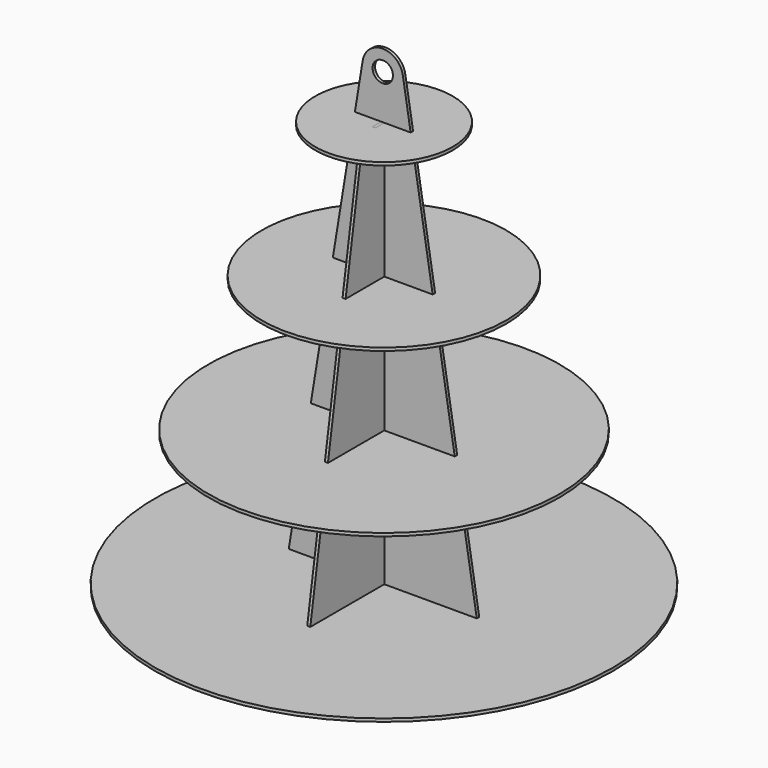
from build123d import *

# Parameters (mm, degrees)
F0_R      = 10
F1_DEPTH  = 1.5
F2_W      = 3
F2_H      = 220
F3_DEPTH  = 25
F5_DEPTH  = 1.5
F6_W      = 3
F6_H      = 212
F7_DEPTH  = 12.5
F9_R      = 225
F10_DEPTH = 3
F12_R     = 172.5
F13_DEPTH = 3
F15_R     = 120
F16_DEPTH = 3
F18_R     = 67.5
F19_DEPTH = 3


with BuildPart() as f1:
    # F0 (on Front) → F1 (new body, symmetric)
    with BuildSketch(Plane.XZ):
        with BuildLine():
            Line((-92.3427922293, 30), (-195, 30))
            add(Edge.make_bspline(
                [(-195, 30), (-195, 16.186110581), (-168.2676257137, 15.093790554), (-141.795995516, 15.0074163979)],
                knots=[0, 0, 0, 0, 56.9561251752, 56.9561251752, 56.9561251752, 56.9561251752], degree=3))
            ThreePointArc((-141.795995516, 15.0074163979), (-137.776195244, 12.9586763901), (-137.0427819368, 8.5069087898))
            Line((-137.0427819368, 8.5069087898), (-139.3101033649, 1.3001068448))
            ThreePointArc((-139.3101033649, 1.3001068448), (-139.1624566765, 0.4084371736), (-138.3561977712, 0))
            Line((-138.3561977712, 0), (0, 0))
            Line((0, 0), (138.3561977712, 0))
            ThreePointArc((138.3561977712, 0), (139.1624566765, 0.4084371736), (139.3101033649, 1.3001068448))
            Line((139.3101033649, 1.3001068448), (137.0427819368, 8.5069087898))
            ThreePointArc((137.0427819368, 8.5069087898), (137.776195244, 12.9586763901), (141.795995516, 15.0074163979))
            add(Edge.make_bspline(
                [(195, 30), (195, 16.186110581), (168.2676257137, 15.093790554), (141.795995516, 15.0074163979)],
                knots=[0, 0, 0, 0, 56.9561251752, 56.9561251752, 56.9561251752, 56.9561251752], degree=3))
            Line((195, 30), (92.3427922293, 30))
            Line((92.3427922293, 30), (92.3427922293, 33))
            Line((92.3427922293, 33), (74.5588604965, 142.1962788761))
            ThreePointArc((74.5588604965, 142.1962788761), (75.6847331024, 146.2389345764), (79.4938409783, 148))
            Line((79.4938409783, 148), (82.5, 148))
            add(Edge.make_bspline(
                [(142.5, 163), (142.5, 151.0542502936), (110.9798626697, 148), (82.5, 148)],
                knots=[0, 0, 0, 0, 61.8465843843, 61.8465843843, 61.8465843843, 61.8465843843], degree=3))
            Line((142.5, 163), (70.6821372619, 163))
            Line((70.6821372619, 163), (70.6821372619, 166))
            Line((70.6821372619, 166), (52.7101309279, 276.3510879995))
            ThreePointArc((52.7101309279, 276.3510879995), (53.6868072822, 280.2096132801), (57.1717998525, 282.1323563276))
            add(Edge.make_bspline(
                [(90, 296), (90, 287.8812796125), (75.4408356741, 283.8695464407), (57.1717998525, 282.1323563276)],
                knots=[0, 0, 0, 0, 42.0329521278, 42.0329521278, 42.0329521278, 42.0329521278], degree=3))
            Line((90, 296), (49.0214822946, 296))
            Line((49.0214822946, 296), (49.0214822946, 299))
            Line((49.0214822946, 299), (29.5550758212, 418.5269517407))
            ThreePointArc((29.5550758212, 418.5269517407), (30.0968650968, 421.7181131313), (32.479761139, 423.9087416009))
            add(Edge.make_bspline(
                [(32.479761139, 423.9087416009), (25.3871356607, 420.7942687696), (11.9619410008, 419.2400986089), (0, 418.4677997632)],
                knots=[10.6465175628, 10.6465175628, 10.6465175628, 10.6465175628, 34.8130753377, 34.8130753377, 34.8130753377, 34.8130753377], degree=3))
            add(Edge.make_bspline(
                [(-32.479761139, 423.9087416009), (-25.3871356607, 420.7942687696), (-11.9619410008, 419.2400986089), (0, 418.4677997632)],
                knots=[10.6465175628, 10.6465175628, 10.6465175628, 10.6465175628, 34.8130753377, 34.8130753377, 34.8130753377, 34.8130753377], degree=3))
            ThreePointArc((-32.479761139, 423.9087416009), (-30.0968650968, 421.7181131313), (-29.5550758212, 418.5269517407))
            Line((-29.5550758212, 418.5269517407), (-49.0214822946, 299))
            Line((-49.0214822946, 299), (-49.0214822946, 296))
            Line((-49.0214822946, 296), (-90, 296))
            add(Edge.make_bspline(
                [(-90, 296), (-90, 287.8812796125), (-75.4408356741, 283.8695464407), (-57.1717998525, 282.1323563276)],
                knots=[0, 0, 0, 0, 42.0329521278, 42.0329521278, 42.0329521278, 42.0329521278], degree=3))
            ThreePointArc((-57.1717998525, 282.1323563276), (-53.6868072822, 280.2096132801), (-52.7101309279, 276.3510879995))
            Line((-52.7101309279, 276.3510879995), (-70.6821372619, 166))
            Line((-70.6821372619, 166), (-70.6821372619, 163))
            Line((-70.6821372619, 163), (-142.5, 163))
            add(Edge.make_bspline(
                [(-142.5, 163), (-142.5, 151.0542502936), (-110.9798626697, 148), (-82.5, 148)],
                knots=[0, 0, 0, 0, 61.8465843843, 61.8465843843, 61.8465843843, 61.8465843843], degree=3))
            Line((-82.5, 148), (-79.4938409783, 148))
            ThreePointArc((-79.4938409783, 148), (-75.6847331024, 146.2389345764), (-74.5588604965, 142.1962788761))
            Line((-74.5588604965, 142.1962788761), (-92.3427922293, 33))
            Line((-92.3427922293, 33), (-92.3427922293, 30))
        make_face()
        with BuildLine():
            add(Edge.make_bspline(
                [(-37.5, 429), (-37.5, 426.955715158), (-35.6043998411, 425.2808149431), (-32.479761139, 423.9087416009)],
                knots=[0, 0, 0, 0, 10.6465175628, 10.6465175628, 10.6465175628, 10.6465175628], degree=3))
            add(Edge.make_bspline(
                [(-32.479761139, 423.9087416009), (-25.3871356607, 420.7942687696), (-11.9619410008, 419.2400986089), (0, 418.4677997632)],
                knots=[10.6465175628, 10.6465175628, 10.6465175628, 10.6465175628, 34.8130753377, 34.8130753377, 34.8130753377, 34.8130753377], degree=3))
            add(Edge.make_bspline(
                [(32.479761139, 423.9087416009), (25.3871356607, 420.7942687696), (11.9619410008, 419.2400986089), (0, 418.4677997632)],
                knots=[10.6465175628, 10.6465175628, 10.6465175628, 10.6465175628, 34.8130753377, 34.8130753377, 34.8130753377, 34.8130753377], degree=3))
            add(Edge.make_bspline(
                [(37.5, 429), (37.5, 426.955715158), (35.6043998411, 425.2808149431), (32.479761139, 423.9087416009)],
                knots=[0, 0, 0, 0, 10.6465175628, 10.6465175628, 10.6465175628, 10.6465175628], degree=3))
            Line((37.5, 429), (27.3608273272, 429))
            Line((27.3608273272, 429), (27.3608273272, 432))
            Line((27.3608273272, 432), (19.7399219269, 478.793618188))
            ThreePointArc((19.7399219269, 478.793618188), (0, 495.5787336922), (-19.7399219269, 478.793618188))
            Line((-19.7399219269, 478.793618188), (-27.3608273272, 432))
            Line((-27.3608273272, 432), (-27.3608273272, 429))
            Line((-27.3608273272, 429), (-37.5, 429))
        make_face()
        with Locations((0, 475.5787336922)):
            Circle(F0_R, mode=Mode.SUBTRACT)
    extrude(amount=F1_DEPTH, both=True)

    # F2 (on face) → F3 (cut)
    with BuildSketch(Plane.XZ.offset(1.5)):
        with Locations((0, 110)):
            Rectangle(F2_W, F2_H)
    extrude(amount=-F3_DEPTH, mode=Mode.SUBTRACT)


with BuildPart() as f5:
    # F4 (on Right) → F5 (new body, symmetric)
    with BuildSketch(Plane.YZ):
        with BuildLine():
            Line((-92.3427922293, 30), (-195, 30))
            add(Edge.make_bspline(
                [(-195, 30), (-195, 16.335147151), (-168.5112592434, 15.1188411943), (-142.5647102575, 15.0105780321)],
                knots=[0, 0, 0, 0, 56.3416316551, 56.3416316551, 56.3416316551, 56.3416316551], degree=3))
            ThreePointArc((-142.5647102575, 15.0105780321), (-138.4043979513, 12.7524780168), (-137.991624861, 8.0368834052))
            Line((-137.991624861, 8.0368834052), (-140.631448797, 1.8925963671))
            ThreePointArc((-140.631448797, 1.8925963671), (-140.5487271046, 0.9492227505), (-139.7162225162, 0.4978550853))
            Line((-139.7162225162, 0.4978550853), (0, 0))
            Line((0, 0), (139.7162225162, 0.4978550853))
            ThreePointArc((139.7162225162, 0.4978550853), (140.5487271046, 0.9492227505), (140.631448797, 1.8925963671))
            Line((140.631448797, 1.8925963671), (137.991624861, 8.0368834052))
            ThreePointArc((137.991624861, 8.0368834052), (138.4043979513, 12.7524780168), (142.5647102575, 15.0105780321))
            add(Edge.make_bspline(
                [(195, 30), (195, 16.335147151), (168.5112592434, 15.1188411943), (142.5647102575, 15.0105780321)],
                knots=[0, 0, 0, 0, 56.3416316551, 56.3416316551, 56.3416316551, 56.3416316551], degree=3))
            Line((195, 30), (92.3427922293, 30))
            Line((92.3427922293, 30), (92.3427922293, 33))
            Line((92.3427922293, 33), (74.5588604965, 142.1962788761))
            ThreePointArc((74.5588604965, 142.1962788761), (75.6847331024, 146.2389345764), (79.4938409783, 148))
            Line((79.4938409783, 148), (82.5, 148))
            add(Edge.make_bspline(
                [(142.5, 163), (142.5, 151.0542502936), (110.9798626697, 148), (82.5, 148)],
                knots=[0, 0, 0, 0, 61.8465843843, 61.8465843843, 61.8465843843, 61.8465843843], degree=3))
            Line((142.5, 163), (70.6821372619, 163))
            Line((70.6821372619, 163), (70.6821372619, 166))
            Line((70.6821372619, 166), (52.7101309279, 276.3510879995))
            ThreePointArc((52.7101309279, 276.3510879995), (53.6868072822, 280.2096132801), (57.1717998525, 282.1323563276))
            add(Edge.make_bspline(
                [(90, 296), (90, 287.8812796125), (75.4408356741, 283.8695464407), (57.1717998525, 282.1323563276)],
                knots=[0, 0, 0, 0, 42.0329521278, 42.0329521278, 42.0329521278, 42.0329521278], degree=3))
            Line((90, 296), (49.0214822946, 296))
            Line((49.0214822946, 296), (49.0214822946, 299))
            Line((49.0214822946, 299), (29.5550758212, 418.5269517407))
            ThreePointArc((29.5550758212, 418.5269517407), (30.0968650968, 421.7181131313), (32.479761139, 423.9087416009))
            add(Edge.make_bspline(
                [(32.479761139, 423.9087416009), (25.3871356607, 420.7942687696), (11.9619410008, 419.2400986089), (0, 418.4677997632)],
                knots=[10.6465175628, 10.6465175628, 10.6465175628, 10.6465175628, 34.8130753377, 34.8130753377, 34.8130753377, 34.8130753377], degree=3))
            add(Edge.make_bspline(
                [(-32.479761139, 423.9087416009), (-25.3871356607, 420.7942687696), (-11.9619410008, 419.2400986089), (0, 418.4677997632)],
                knots=[10.6465175628, 10.6465175628, 10.6465175628, 10.6465175628, 34.8130753377, 34.8130753377, 34.8130753377, 34.8130753377], degree=3))
            ThreePointArc((-32.479761139, 423.9087416009), (-30.0968650968, 421.7181131313), (-29.5550758212, 418.5269517407))
            Line((-29.5550758212, 418.5269517407), (-49.0214822946, 299))
            Line((-49.0214822946, 299), (-49.0214822946, 296))
            Line((-49.0214822946, 296), (-90, 296))
            add(Edge.make_bspline(
                [(-90, 296), (-90, 287.8812796125), (-75.4408356741, 283.8695464407), (-57.1717998525, 282.1323563276)],
                knots=[0, 0, 0, 0, 42.0329521278, 42.0329521278, 42.0329521278, 42.0329521278], degree=3))
            ThreePointArc((-57.1717998525, 282.1323563276), (-53.6868072822, 280.2096132801), (-52.7101309279, 276.3510879995))
            Line((-52.7101309279, 276.3510879995), (-70.6821372619, 166))
            Line((-70.6821372619, 166), (-70.6821372619, 163))
            Line((-70.6821372619, 163), (-142.5, 163))
            add(Edge.make_bspline(
                [(-142.5, 163), (-142.5, 151.0542502936), (-110.9798626697, 148), (-82.5, 148)],
                knots=[0, 0, 0, 0, 61.8465843843, 61.8465843843, 61.8465843843, 61.8465843843], degree=3))
            Line((-82.5, 148), (-79.4938409783, 148))
            ThreePointArc((-79.4938409783, 148), (-75.6847331024, 146.2389345764), (-74.5588604965, 142.1962788761))
            Line((-74.5588604965, 142.1962788761), (-92.3427922293, 33))
            Line((-92.3427922293, 33), (-92.3427922293, 30))
        make_face()
        with BuildLine():
            add(Edge.make_bspline(
                [(-37.5, 429), (-37.5, 426.955715158), (-35.6043998411, 425.2808149431), (-32.479761139, 423.9087416009)],
                knots=[0, 0, 0, 0, 10.6465175628, 10.6465175628, 10.6465175628, 10.6465175628], degree=3))
            add(Edge.make_bspline(
                [(-32.479761139, 423.9087416009), (-25.3871356607, 420.7942687696), (-11.9619410008, 419.2400986089), (0, 418.4677997632)],
                knots=[10.6465175628, 10.6465175628, 10.6465175628, 10.6465175628, 34.8130753377, 34.8130753377, 34.8130753377, 34.8130753377], degree=3))
            add(Edge.make_bspline(
                [(32.479761139, 423.9087416009), (25.3871356607, 420.7942687696), (11.9619410008, 419.2400986089), (0, 418.4677997632)],
                knots=[10.6465175628, 10.6465175628, 10.6465175628, 10.6465175628, 34.8130753377, 34.8130753377, 34.8130753377, 34.8130753377], degree=3))
            add(Edge.make_bspline(
                [(37.5, 429), (37.5, 426.955715158), (35.6043998411, 425.2808149431), (32.479761139, 423.9087416009)],
                knots=[0, 0, 0, 0, 10.6465175628, 10.6465175628, 10.6465175628, 10.6465175628], degree=3))
            Line((37.5, 429), (12.5, 429))
            Line((12.5, 429), (12.5, 432))
            Line((12.5, 432), (-12.5, 432))
            Line((-12.5, 432), (-12.5, 429))
            Line((-12.5, 429), (-37.5, 429))
        make_face()
    extrude(amount=F5_DEPTH, both=True)

    # F6 (on face) → F7 (cut, symmetric)
    with BuildSketch(Plane(origin=(-1.5, 0, 0), x_dir=(0, -1, 0), z_dir=(-1, 0, 0))):
        with Locations((0, 326)):
            Rectangle(F6_W, F6_H)
    extrude(amount=F7_DEPTH, both=True, mode=Mode.SUBTRACT)


with BuildPart() as f10:
    # F9 (on plane+point) → F10 (new body)
    with BuildSketch(Plane.XY.offset(30)):
        Circle(F9_R)
        Polygon((-1.5, -1.5), (-92.3427922293, -1.5), (-92.3427922293, 1.5), (-1.5, 1.5), (-1.5, 92.3427922293), (1.5, 92.3427922293), (1.5, 1.5), (92.3427922293, 1.5), (92.3427922293, -1.5), (1.5, -1.5), (1.5, -92.3427922293), (-1.5, -92.3427922293), align=None, mode=Mode.SUBTRACT)
    extrude(amount=F10_DEPTH)


with BuildPart() as f13:
    # F12 (on plane+point) → F13 (new body)
    with BuildSketch(Plane.XY.offset(163)):
        Circle(F12_R)
        Polygon((1.5, -1.5), (1.5, -70.6821372619), (-1.5, -70.6821372619), (-1.5, -1.5), (-70.6821372619, -1.5), (-70.6821372619, 1.5), (-1.5, 1.5), (-1.5, 70.6821372619), (1.5, 70.6821372619), (1.5, 1.5), (70.6821372619, 1.5), (70.6821372619, -1.5), align=None, mode=Mode.SUBTRACT)
    extrude(amount=F13_DEPTH)


with BuildPart() as f16:
    # F15 (on plane+point) → F16 (new body)
    with BuildSketch(Plane.XY.offset(296)):
        Circle(F15_R)
        Polygon((1.5, -1.5), (1.5, -49.0214822946), (-1.5, -49.0214822946), (-1.5, -1.5), (-49.0214822946, -1.5), (-49.0214822946, 1.5), (-1.5, 1.5), (-1.5, 49.0214822946), (1.5, 49.0214822946), (1.5, 1.5), (49.0214822946, 1.5), (49.0214822946, -1.5), align=None, mode=Mode.SUBTRACT)
    extrude(amount=F16_DEPTH)


with BuildPart() as f19:
    # F18 (on plane+point) → F19 (new body)
    with BuildSketch(Plane.XY.offset(429)):
        Circle(F18_R)
        Polygon((-1.5, -1.5), (-27.3608273272, -1.5), (-27.3608273272, 1.5), (-1.5, 1.5), (-1.5, 12.5), (1.5, 12.5), (1.5, 1.5), (27.3608273272, 1.5), (27.3608273272, -1.5), (1.5, -1.5), (1.5, -12.5), (-1.5, -12.5), align=None, mode=Mode.SUBTRACT)
    extrude(amount=F19_DEPTH)


solid = Compound([f1.part, f5.part, f10.part, f13.part, f16.part, f19.part])
